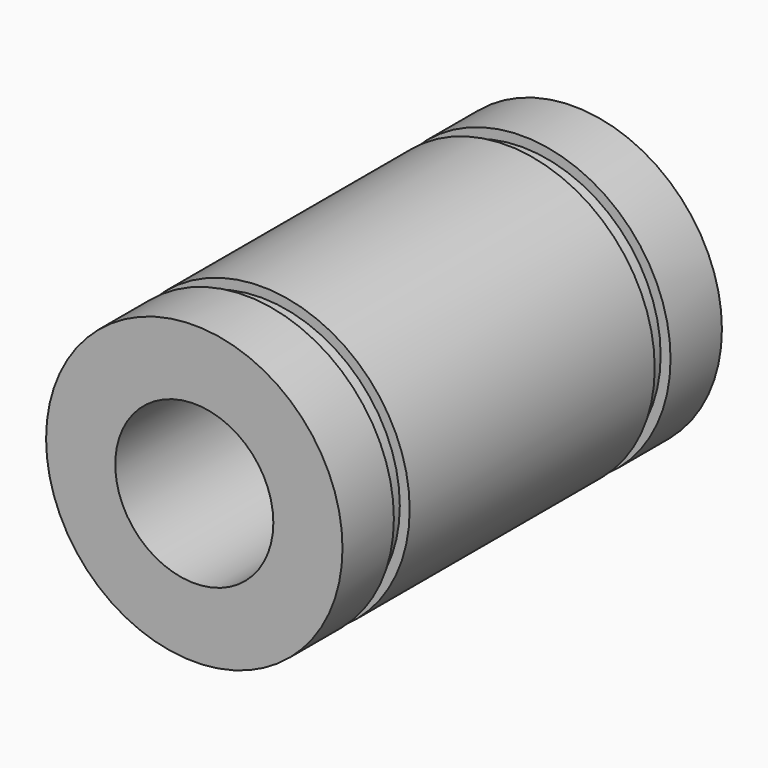
from build123d import *

# Parameters (mm, degrees)
F0_R     = 7.5
F0_R_2   = 4
F1_DEPTH = 3.25
F2_R     = 7
F2_R_2   = 4
F3_DEPTH = 1
F4_R     = 7.5
F4_R_2   = 7
F4_R_3   = 4
F5_DEPTH = 15.5
F6_R     = 7
F6_R_2   = 4
F7_DEPTH = 1
F8_R     = 7.5
F8_R_2   = 7
F8_R_3   = 4
F9_DEPTH = 3.25


# Not quite as in the source:
# - a feature names something its author has since deleted; it is built from what else it names


with BuildPart() as f1:
    # F0 (on Front) → F1 (new body)
    with BuildSketch(Plane.XZ):
        Circle(F0_R)
        Circle(F0_R_2, mode=Mode.SUBTRACT)
    extrude(amount=F1_DEPTH)

    # F2 (on face) → F3 (join)
    with BuildSketch(Plane.XZ.offset(3.25)):
        Circle(F2_R)
        Circle(F2_R_2, mode=Mode.SUBTRACT)
    extrude(amount=F3_DEPTH)

    # F4 (on face) → F5 (join)
    with BuildSketch(Plane.XZ.offset(4.25)):
        Circle(F4_R)
        Circle(F4_R_2, mode=Mode.SUBTRACT)
        Circle(F4_R_2)
        Circle(F4_R_3, mode=Mode.SUBTRACT)
    extrude(amount=F5_DEPTH)

    # F6 (on face) → F7 (join)
    with BuildSketch(Plane.XZ.offset(19.75)):
        Circle(F6_R)
        Circle(F6_R_2, mode=Mode.SUBTRACT)
    extrude(amount=F7_DEPTH)

    # F8 (on face) → F9 (join)
    with BuildSketch(Plane.XZ.offset(20.75)):
        Circle(F8_R)
        Circle(F8_R_2, mode=Mode.SUBTRACT)
        Circle(F8_R_2)
        Circle(F8_R_3, mode=Mode.SUBTRACT)
    extrude(amount=F9_DEPTH)


solid = f1.part
